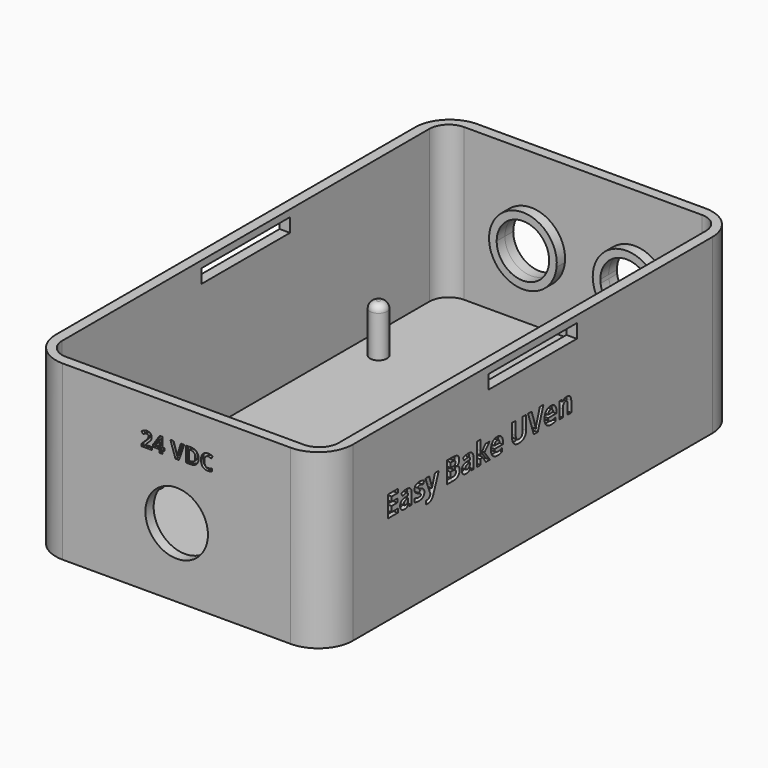
from build123d import *

# Parameters (mm, degrees)
F1_DEPTH      = 31.75
F4_DEPTH      = 27.94
F6_R          = 1.5494
F7_DEPTH      = 8.89
F6_R_2        = 1.543314
F6_R_3        = 1.565784
F6_R_4        = 1.561471
F8_R          = 1.27
F8_2_R        = 1.27
F8_3_R        = 1.27
F8_4_R        = 1.27
F10_DEPTH     = 11.43
F11_DEPTH     = 3.81
F12_R         = 5.75
F13_DEPTH     = 3.81
F16_DEPTH     = 54.611
F17_TEXT_SIZE = 3.892297
F18_DEPTH     = 0.5
F19_TEXT_SIZE = 5.449212
F20_DEPTH     = 0.85


# Not quite as in the source:
# - Text() gives the source's letters only with a copy of the font that has no kerning and outlines rounded to 1/6400 em; it was checked with that copy


with BuildPart() as f1:
    # F0 (on Top) → F1 (new body)
    with BuildSketch(Plane.XY):
        with BuildLine():
            Line((-20.955, -47.625), (20.955, -47.625))
            ThreePointArc((20.955, -47.625), (25.445128, -45.765128), (27.305, -41.275))
            Line((27.305, -41.275), (27.305, 41.275))
            ThreePointArc((27.305, 41.275), (25.445128, 45.765128), (20.955, 47.625))
            Line((20.955, 47.625), (-20.955, 47.625))
            ThreePointArc((-20.955, 47.625), (-25.445128, 45.765128), (-27.305, 41.275))
            Line((-27.305, 41.275), (-27.305, -41.275))
            ThreePointArc((-27.305, -41.275), (-25.445128, -45.765128), (-20.955, -47.625))
        make_face()
    extrude(amount=F1_DEPTH)

    # F3 (on face) → F4 (cut)
    with BuildSketch(Plane.XY.offset(31.75)):
        with BuildLine():
            Line((21.844, 45.72), (-21.844, 45.72))
            ThreePointArc((-21.844, 45.72), (-24.358472, 44.678472), (-25.4, 42.164))
            Line((-25.4, 42.164), (-25.4, -42.164))
            ThreePointArc((-25.4, -42.164), (-24.358472, -44.678472), (-21.844, -45.72))
            Line((-21.844, -45.72), (21.844, -45.72))
            ThreePointArc((21.844, -45.72), (24.358472, -44.678472), (25.4, -42.164))
            Line((25.4, -42.164), (25.4, 42.164))
            ThreePointArc((25.4, 42.164), (24.358472, 44.678472), (21.844, 45.72))
        make_face()
    extrude(amount=-F4_DEPTH, mode=Mode.SUBTRACT)

    # F9 (on face) → F10 (cut)
    with BuildSketch(Plane(origin=(0, 47.625, 0), x_dir=(-1, 0, 0), z_dir=(0, 1, 0))):
        with BuildLine():
            ThreePointArc((-4.699, 16.509995), (-14.340499, 16.828185), (-4.740958, 15.875))
            ThreePointArc((-4.740958, 15.875), (-4.709501, 16.191805), (-4.699, 16.509995))
        make_face()
        with BuildLine():
            ThreePointArc((14.351, 16.509995), (9.20681, 21.325494), (4.740958, 15.875))
            ThreePointArc((4.740958, 15.875), (9.84319, 11.694496), (14.351, 16.509995))
        make_face()
    extrude(amount=-F10_DEPTH, mode=Mode.SUBTRACT)

    # F9 (on face) → F11 (join)
    with BuildSketch(Plane(origin=(0, 47.625, 0), x_dir=(-1, 0, 0), z_dir=(0, 1, 0))):
        with BuildLine():
            ThreePointArc((-3.305921, 16.509995), (-15.735948, 16.827908), (-3.338424, 15.875))
            ThreePointArc((-3.338424, 15.875), (-3.314052, 16.192082), (-3.305921, 16.509995))
        make_face()
        with BuildLine():
            ThreePointArc((-4.699, 16.509995), (-4.709501, 16.191805), (-4.740958, 15.875))
            ThreePointArc((-4.740958, 15.875), (-14.340499, 16.828185), (-4.699, 16.509995))
        make_face(mode=Mode.SUBTRACT)
        with BuildLine():
            ThreePointArc((15.748, 16.509995), (9.207087, 22.724869), (3.334482, 15.875))
            ThreePointArc((3.334482, 15.875), (9.842912, 10.295121), (15.748, 16.509995))
        make_face()
        with BuildLine():
            ThreePointArc((14.351, 16.509995), (9.84319, 11.694496), (4.740958, 15.875))
            ThreePointArc((4.740958, 15.875), (9.20681, 21.325494), (14.351, 16.509995))
        make_face(mode=Mode.SUBTRACT)
    extrude(amount=-F11_DEPTH)

    # F12 (on face) → F13 (cut)
    with BuildSketch(Plane.XZ.offset(47.625)):
        with Locations((0, 12.71335)):
            Circle(F12_R)
    extrude(amount=-F13_DEPTH, mode=Mode.SUBTRACT)

    # F15 (on face) → F16 (cut, through all)
    with BuildSketch(Plane.YZ.offset(27.305)):
        Polygon((10.16, 30.48), (0, 30.48), (-10.16, 30.48), (-10.16, 27.94), (10.16, 27.94), align=None)
    extrude(amount=-F16_DEPTH, mode=Mode.SUBTRACT)

    # F17 (on face) → F18 (cut)
    with BuildSketch(Plane.XZ.offset(47.625)):
        with Locations((-6.616195, 23.067893)):
            Text('24 VDC', F17_TEXT_SIZE, font='Open Sans', font_style=FontStyle.BOLD, text_align=(TextAlign.LEFT, TextAlign.BOTTOM))
    extrude(amount=-F18_DEPTH, mode=Mode.SUBTRACT)

    # F19 (on face) → F20 (cut)
    with BuildSketch(Plane.YZ.offset(27.305)):
        with Locations((-33.699483, 16.499102)):
            Text('Easy Bake UVen', F19_TEXT_SIZE, font='Open Sans', font_style=FontStyle.BOLD, text_align=(TextAlign.LEFT, TextAlign.BOTTOM))
    extrude(amount=-F20_DEPTH, mode=Mode.SUBTRACT)


with BuildPart() as f7:
    # F6 (on face) → F7 (new body)
    with BuildSketch(Plane.XY.offset(3.81)):
        with Locations((20.792063, 21.952555)):
            Circle(F6_R)
    extrude(amount=F7_DEPTH)

    # F8
    f8_edges = [f7.edges().sort_by_distance(p)[0] for p in [
        (19.242663, 21.952555, 12.7),
    ]]
    fillet(f8_edges, radius=F8_R)


with BuildPart() as f7b:
    # F6 (on face) → F7, piece 2 (new body)
    with BuildSketch(Plane.XY.offset(3.81)):
        with Locations((20.672349, -29.57597)):
            Circle(F6_R_2)
    extrude(amount=F7_DEPTH)

    # F8#2
    f8_2_edges = [f7b.edges().sort_by_distance(p)[0] for p in [
        (19.129036, -29.57597, 12.7),
    ]]
    fillet(f8_2_edges, radius=F8_2_R)


with BuildPart() as f7c:
    # F6 (on face) → F7, piece 3 (new body)
    with BuildSketch(Plane.XY.offset(3.81)):
        with Locations((-20.668013, -29.59623)):
            Circle(F6_R_3)
    extrude(amount=F7_DEPTH)

    # F8#3
    f8_3_edges = [f7c.edges().sort_by_distance(p)[0] for p in [
        (-22.233797, -29.59623, 12.7),
    ]]
    fillet(f8_3_edges, radius=F8_3_R)


with BuildPart() as f7d:
    # F6 (on face) → F7, piece 4 (new body)
    with BuildSketch(Plane.XY.offset(3.81)):
        with Locations((-20.631289, 21.999203)):
            Circle(F6_R_4)
    extrude(amount=F7_DEPTH)

    # F8#4
    f8_4_edges = [f7d.edges().sort_by_distance(p)[0] for p in [
        (-22.19276, 21.999203, 12.7),
    ]]
    fillet(f8_4_edges, radius=F8_4_R)


with BuildPart() as f7c_1:
    # F14: moved
    add(f7c.part.moved(Location((0, 2.54, 0))))


with BuildPart() as f7b_1:
    # F14: moved
    add(f7b.part.moved(Location((0, 2.54, 0))))


with BuildPart() as f7_1:
    # F14: moved
    add(f7.part.moved(Location((0, 2.54, 0))))


with BuildPart() as f7d_1:
    # F14: moved
    add(f7d.part.moved(Location((0, 2.54, 0))))


solid = Compound([f1.part, f7c_1.part, f7b_1.part, f7_1.part, f7d_1.part])
